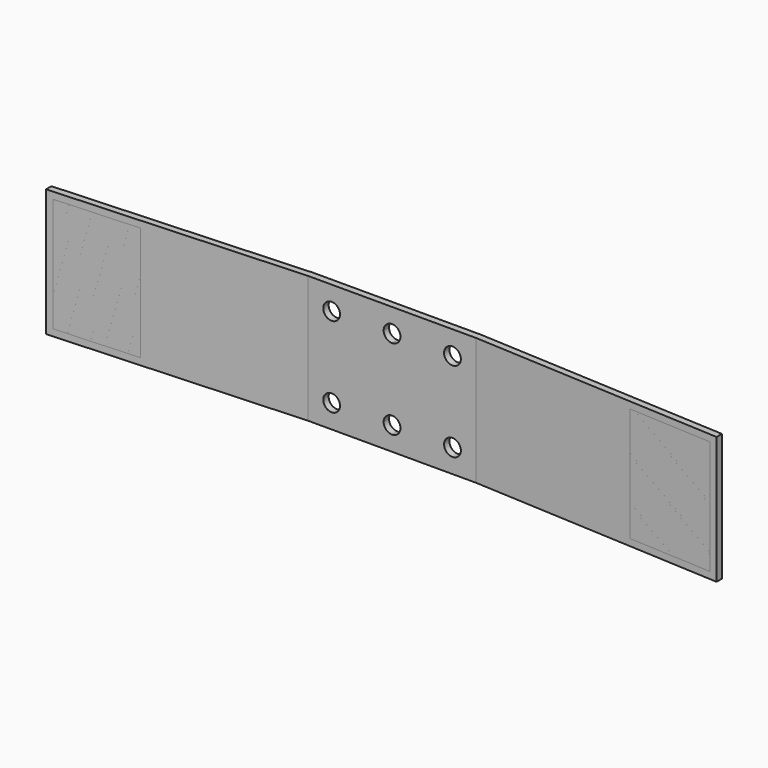
from build123d import *

# Parameters (mm, degrees)
F1_DEPTH = 38
F3_W     = 25
F3_H     = 34
F4_DEPTH = 3.5
F2_R     = 2.5
F6_DEPTH = 25


with BuildPart() as f1:
    # F0 (on Top) → F1 (new body)
    with BuildSketch(Plane.XY):
        Polygon((0, -2), (0, 0), (-25, 0), (-99.8932573734, -4), (-99.8932573734, -6), (-25, -2), align=None)
        Polygon((25, 0), (0, 0), (0, -2), (25, -2), (99.8932573734, -6), (99.8932573734, -4), align=None)
    extrude(amount=F1_DEPTH)

    # F2 (on face) → F6 (cut)
    with BuildSketch(Plane(origin=(0, 0, 0), x_dir=(-1, 0, 0), z_dir=(0, 1, 0))):
        with BuildLine():
            ThreePointArc((2.5, 31), (1.767766953, 32.767766953), (0, 33.5))
            Line((0, 33.5), (0, 28.5))
            ThreePointArc((0, 28.5), (1.767766953, 29.232233047), (2.5, 31))
        make_face()
        with BuildLine():
            ThreePointArc((2.5, 7), (1.767766953, 8.767766953), (0, 9.5))
            Line((0, 9.5), (0, 4.5))
            ThreePointArc((0, 4.5), (1.767766953, 5.232233047), (2.5, 7))
        make_face()
        with BuildLine():
            Line((0, 4.5), (0, 9.5))
            ThreePointArc((0, 9.5), (-2.5, 7), (0, 4.5))
        make_face()
        with BuildLine():
            Line((0, 28.5), (0, 33.5))
            ThreePointArc((0, 33.5), (-2.5, 31), (0, 28.5))
        make_face()
        with Locations((18, 31)):
            Circle(F2_R)
        with Locations((18, 7)):
            Circle(F2_R)
        with Locations((-18, 31)):
            Circle(F2_R)
        with Locations((-18, 7)):
            Circle(F2_R)
    extrude(amount=-F6_DEPTH, mode=Mode.SUBTRACT)


with BuildPart() as f4:
    # F3 (on face) → F4 (new body)
    with BuildSketch(Plane(origin=(0.0354037438, -0.6628754245, 0), x_dir=(0.998576765, 0.0533333333, 0), z_dir=(0.0533333333, -0.998576765, 0))):
        with Locations((-85.5710857911, 19)):
            Rectangle(F3_W, F3_H)
    extrude(amount=-F4_DEPTH)


with BuildPart() as f5_1:
    # F5: instance of F4
    add(f4.part.mirror(Plane.YZ))


solid = Compound([f1.part, f4.part, f5_1.part])
